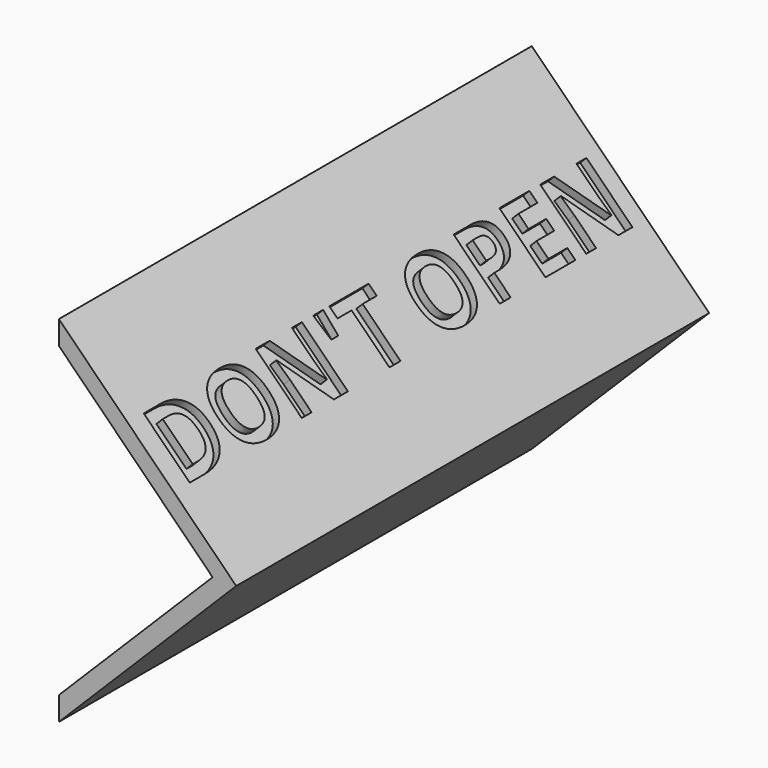
from build123d import *

# Parameters (mm, degrees)
F1_DEPTH     = 5
F3_DEPTH     = 25
F4_TEXT_SIZE = 7.7094887946
F5_DEPTH     = 0.75
F6_R         = 1


# Not quite as in the source:
# - Text() gives the source's letters only with a copy of the font that has no kerning and outlines rounded to 1/6400 em; it was checked with that copy


with BuildPart() as f1:
    # F0 (on Front) → F1 (new body, symmetric)
    with BuildSketch(Plane.XZ):
        with BuildLine():
            ThreePointArc((-4.0150350545, 5.73406431), (7, 0), (-4.0150350545, -5.73406431))
            Line((-4.0150350545, -5.73406431), (-5.7357643635, -8.1915204429))
            ThreePointArc((-5.7357643635, -8.1915204429), (10, 0), (-5.7357643635, 8.1915204429))
            Line((-5.7357643635, 8.1915204429), (-4.0150350545, 5.73406431))
        make_face()
    extrude(amount=F1_DEPTH, both=True)

    # F2 (on Front) → F3 (join, symmetric)
    with BuildSketch(Plane.XZ):
        Polygon((0, 13), (13, 0), (0, -13), (0, -15), (15, 0), (0, 15), align=None)
    extrude(amount=F3_DEPTH, both=True)

    # F4 (on face) → F5 (cut)
    with BuildSketch(Plane(origin=(7.5, 0, 7.5), x_dir=(0.7071067812, 0, -0.7071067812), z_dir=(0.7071067812, 0, 0.7071067812))):
        with Locations(Location((3.1315365242, -24), (0, 0, 90))):
            Text("DON'T OPEN", F4_TEXT_SIZE, font='Open Sans', font_style=FontStyle.BOLD, text_align=(TextAlign.LEFT, TextAlign.BOTTOM))
    extrude(amount=-F5_DEPTH, mode=Mode.SUBTRACT)

    # F6
    f6_edges = [f1.edges().sort_by_distance(p)[0] for p in [
        (-4.015035, 0, 5.734064),
        (-5.735764, 0, 8.19152),
        (-4.015035, 0, -5.734064),
        (-5.735764, 0, -8.19152),
    ]]
    fillet(f6_edges, radius=F6_R)


solid = f1.part
